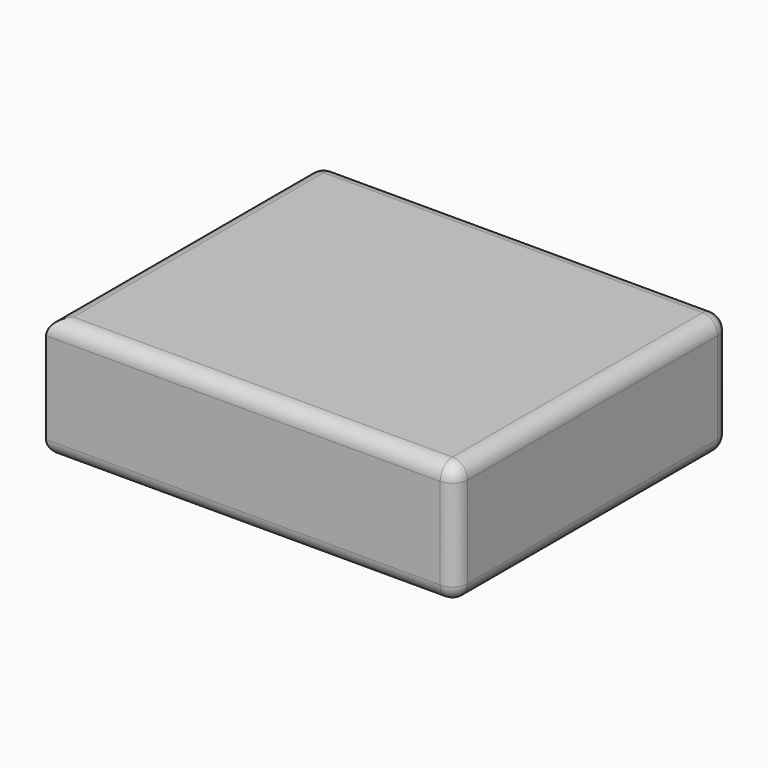
from build123d import *

# Parameters (mm, degrees)
F0_W     = 134.5701217651
F0_H     = 87.3861983418
F1_DEPTH = 40
F2_DEPTH = 25.4
F3_R     = 5


with BuildPart() as f1:
    # F0 (on Top) → F1 (new body)
    with BuildSketch(Plane.XY):
        with Locations((67.2850608826, -43.6930991709)):
            Rectangle(F0_W, F0_H)
    extrude(amount=F1_DEPTH)

    # F2 (add): a face of the model
    f2_faces = [f1.faces().sort_by_distance(p)[0] for p in [
        (67.2850608826, -87.3861983418, 20),
    ]]
    extrude(f2_faces, amount=F2_DEPTH)

    # F3
    f3_edges = [f1.edges().sort_by_distance(p)[0] for p in [
        (134.570122, -56.393099, 40),
        (67.285061, 0, 40),
        (0, -56.393099, 40),
        (67.285061, -112.786198, 40),
        (67.285061, 0, 0),
        (0, -56.393099, 0),
        (67.285061, -112.786198, 0),
        (134.570122, -56.393099, 0),
        (134.570122, 0, 20),
        (134.570122, -112.786198, 20),
        (0, 0, 20),
    ]]
    fillet(f3_edges, radius=F3_R)


solid = f1.part
